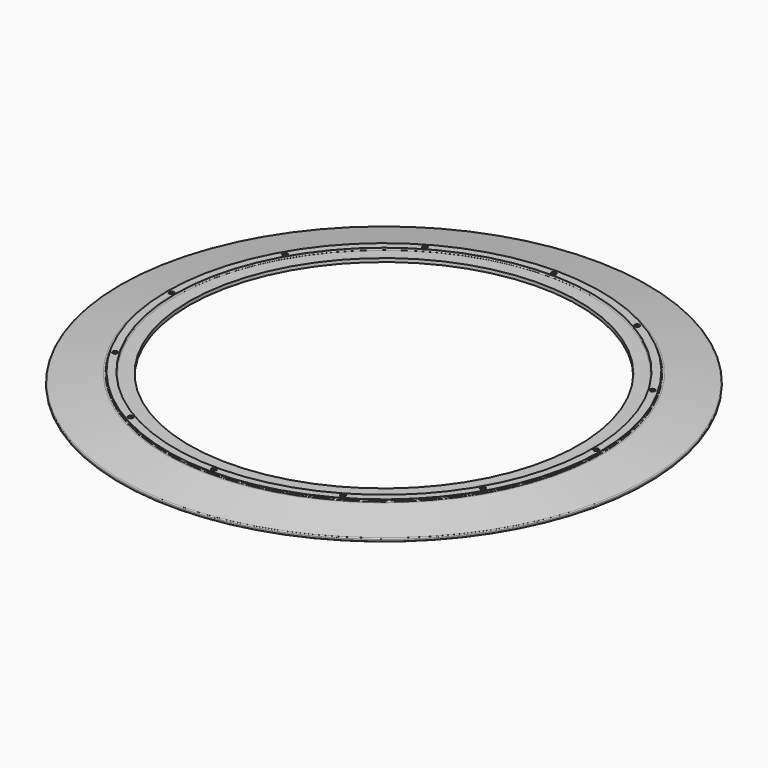
from build123d import *

# Parameters (mm, degrees)
F2_R            = 2
F3_R            = 2
F5_D            = 7
F5_CBORE_D      = 11
F5_CBORE_DEPTH  = 3
F5_COPIES_COUNT = 12


# Not quite as in the source:
# - a pattern or mirror of a feature is missing from the dataset's text; its kind, count and spacing are read off the source's solid


with BuildPart() as f1:
    # F0 (on Front) → F1 (revolve)
    with BuildSketch(Plane.XZ):
        with BuildLine():
            Line((-475, -4), (-475, 0))
            Line((-475, 0), (-492.5, 0))
            Line((-492.5, 0), (-492.5, -4))
            Line((-492.5, -4), (-498.1718563043, -4.1215379759))
            Line((-498.1718563043, -4.1215379759), (-598.3472963553, -21.7851708612))
            ThreePointArc((-598.3472963553, -21.7851708612), (-599.6383040886, -22.6076334946), (-599.969615506, -24.1020827226))
            Line((-599.969615506, -24.1020827226), (-599.3949460194, -28.0049144208))
            ThreePointArc((-599.3949460194, -28.0049144208), (-598.5865316264, -29.3354528156), (-597.0689842363, -29.68318284))
            Line((-597.0689842363, -29.68318284), (-496.782670883, -12))
            Line((-496.782670883, -12), (-442.75, -12))
            Line((-442.75, -12), (-442.75, -4))
            Line((-442.75, -4), (-475, -4))
        make_face()
    revolve(axis=Axis((0, 0, -202.4746355881), (0, 0, -1)))

    # F2
    f2_edges = [f1.edges().sort_by_distance(p)[0] for p in [
        (475, 0, -4),
    ]]
    fillet(f2_edges, radius=F2_R)

    # F3
    f3_edges = [f1.edges().sort_by_distance(p)[0] for p in [
        (492.5, 0, -4),
    ]]
    fillet(f3_edges, radius=F3_R)

    # F5 (through all)
    with Locations(Plane.XY):
        with Locations((482.5, 0)):
            f5 = CounterBoreHole(F5_D / 2, F5_CBORE_D / 2, F5_CBORE_DEPTH)

    # F5_copies: F5 ×12 about axis
    f5_copies_axis = Axis((0, 0, 0), (0, 0, 1))
    for i in range(1, F5_COPIES_COUNT):
        add(f5.rotate(f5_copies_axis, i * 360 / F5_COPIES_COUNT), mode=Mode.SUBTRACT)


solid = f1.part
